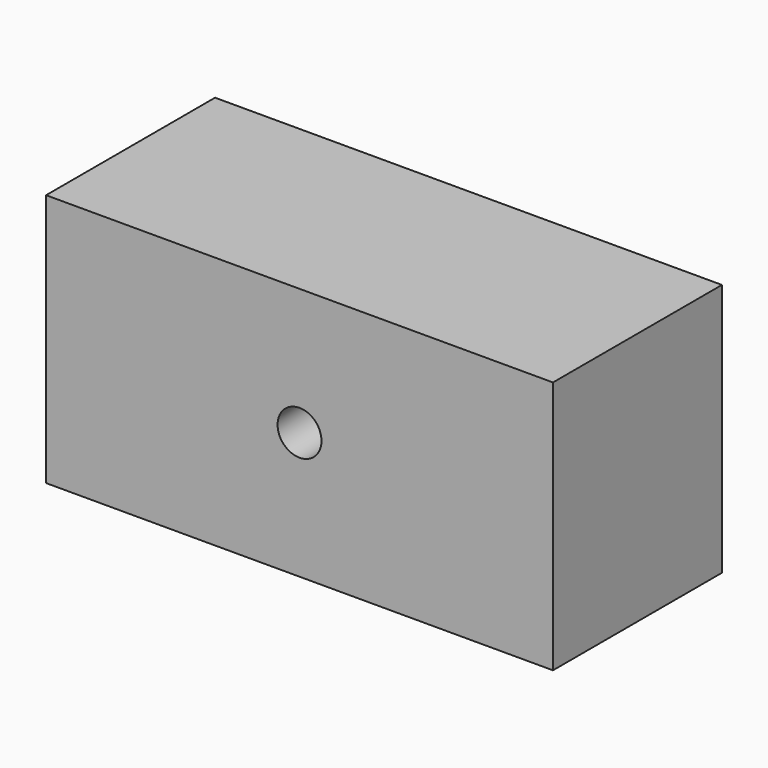
from build123d import *

# Parameters (mm, degrees)
F0_W     = 152.4
F0_H     = 63.5
F1_DEPTH = 76.2
F2_R     = 6.604
F3_DEPTH = 12.7


# Not quite as in the source:
# - a feature names something its author has since deleted; it is built from what else it names


with BuildPart() as f1:
    # F0 (on Top) → F1 (new body)
    with BuildSketch(Plane.XY):
        with Locations((76.2, 31.75)):
            Rectangle(F0_W, F0_H)
    extrude(amount=F1_DEPTH)

    # F2 (on face) → F3 (cut)
    with BuildSketch(Plane.XZ):
        with Locations((76.2, 38.1)):
            Circle(F2_R)
    extrude(amount=-F3_DEPTH, mode=Mode.SUBTRACT)


solid = f1.part
